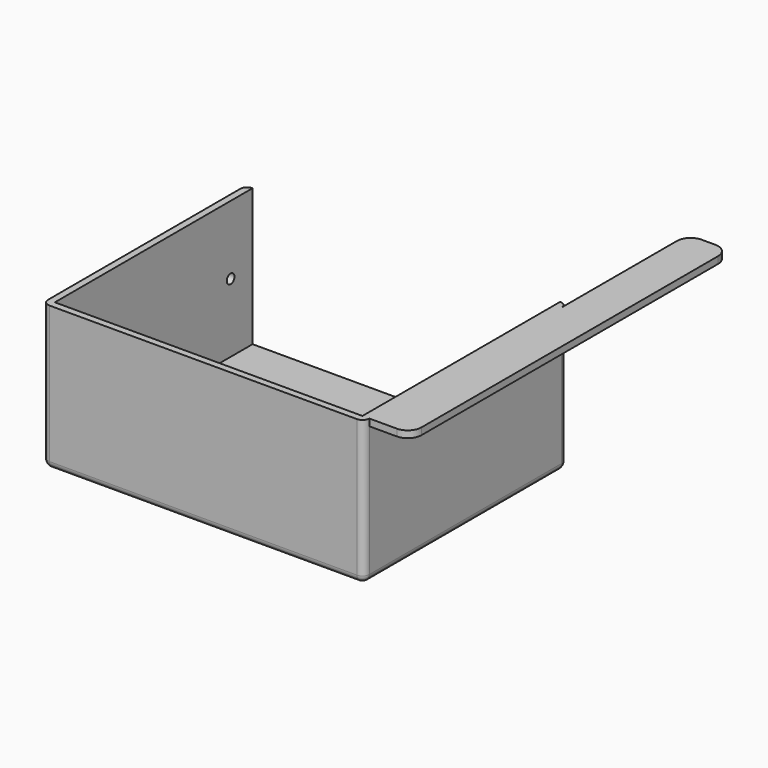
from build123d import *

# Parameters (mm, degrees)
F0_W     = 117
F0_H     = 92.5
F1_DEPTH = 2.5
F2_W     = 2.5
F2_H     = 90
F3_DEPTH = 50
F2_W_2   = 47
F2_H_2   = 28
F4_DEPTH = 25
F5_R     = 1.75
F6_DEPTH = 25
F7_R     = 2.49999
F8_W     = 57.49999
F8_H     = 2.5
F8_W_2   = 87.50001
F9_DEPTH = 15
F10_R    = 5


# Not quite as in the source:
# - a fillet or chamfer is up to 0.001 mm smaller than in the source, because OpenCascade refuses the exact size


with BuildPart() as f1:
    # F0 (on Top) → F1 (new body)
    with BuildSketch(Plane.XY):
        with Locations((0, 6.6284866768)):
            Rectangle(F0_W, F0_H)
    extrude(amount=F1_DEPTH)

    # F2 (on face) → F3 (join)
    with BuildSketch(Plane.XY.offset(2.5)):
        with Locations((57.25, 7.8784866768)):
            Rectangle(F2_W, F2_H)
        Polygon((-58.5, -37.1215133232), (-58.5, -39.6215133232), (58.5, -39.6215133232), (58.5, -37.1215133232), (56, -37.1215133232), (-56, -37.1215133232), align=None)
        with Locations((-57.25, 7.8784866768)):
            Rectangle(F2_W, F2_H)
    extrude(amount=F3_DEPTH)

    # F2 (on face) → F4 (cut)
    with BuildSketch(Plane.XY.offset(2.5)):
        with Locations((-22.5, -15.6215133232)):
            Rectangle(F2_W_2, F2_H_2)
    extrude(amount=-F4_DEPTH, mode=Mode.SUBTRACT)

    # F5 (on face) → F6 (cut)
    with BuildSketch(Plane(origin=(-58.5, 0, 0), x_dir=(0, -1, 0), z_dir=(-1, 0, 0))):
        with Locations((-42.8784866768, 27.5)):
            Circle(F5_R)
    extrude(amount=-F6_DEPTH, mode=Mode.SUBTRACT)

    # F7 (radius 2.5 in the source; OpenCascade refuses exactly that, so slightly less here)
    f7_edges = [f1.edges().sort_by_distance(p)[0] for p in [
        (-58.5, 6.628487, 0),
        (-58.5, -39.621513, 26.25),
        (0, -39.621513, 0),
        (58.5, 6.628487, 0),
        (58.5, -39.621513, 26.25),
        (0, 52.878487, 0),
        (-58.5, 52.878487, 26.25),
        (58.5, 52.878487, 26.25),
    ]]
    fillet(f7_edges, radius=F7_R)

    # F8 (on face) → F9 (join)
    with BuildSketch(Plane.YZ.offset(58.5)):
        with Locations((79.1284916768, 51.25)):
            Rectangle(F8_W, F8_H)
        with Locations((6.6284916768, 51.25)):
            Rectangle(F8_W_2, F8_H)
    extrude(amount=F9_DEPTH)

    # F10
    f10_edges = [f1.edges().sort_by_distance(p)[0] for p in [
        (73.5, 107.878487, 51.25),
        (58.5, 107.878487, 51.25),
        (73.5, -37.121513, 51.25),
    ]]
    fillet(f10_edges, radius=F10_R)


solid = f1.part
